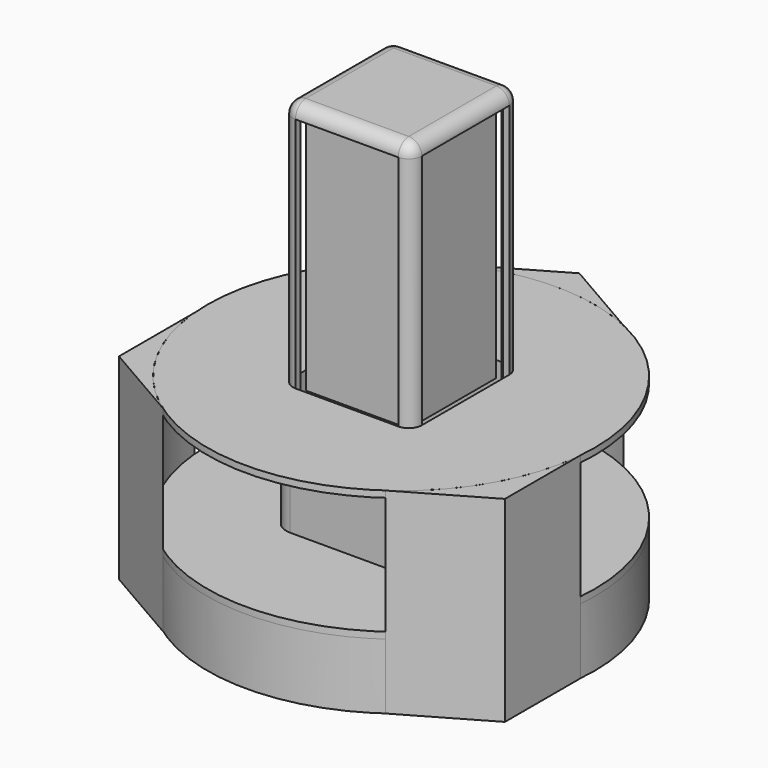
from build123d import *

# Parameters (mm, degrees)
F2_DEPTH     = 76.2
F0_R         = 75.1900139913
F3_DEPTH     = 25.4
F4_W         = 50.0582046807
F4_H         = 52.6002421975
F5_DEPTH     = 147.828
F6_R         = 5.08
F7_DEPTH     = 50.8
F8_T         = -2.54
F9_T         = 2.54
F9_T4_ANGLE  = 90.000000001
F9_T6_ANGLE  = 90.000000001
F9_T8_ANGLE  = 90.000000001
F9_T10_ANGLE = 90.000000001
F10_DEPTH    = 99.822


# Not quite as in the source:
# - a shell that OpenCascade refuses in one call is made with other operations: the cavity is built on its own and cut out


with BuildPart() as f2:
    # F1 (on face) → F2 (new body)
    with BuildSketch(Plane.XY):
        with BuildLine():
            Line((-74.8964771628, -6.6374628139), (-74.8964771628, -43.2415012513))
            Line((-74.8964771628, -43.2415012513), (-43.1964499949, -61.5435204701))
            ThreePointArc((-43.1964499949, -61.5435204701), (-65.1164622274, -37.5950069956), (-74.8964771628, -6.6374628139))
        make_face()
    extrude(amount=F2_DEPTH)


with BuildPart() as f2b:
    # F1 (on face) → F2, piece 2 (new body)
    with BuildSketch(Plane.XY):
        with BuildLine():
            Line((0, 86.4830025026), (-31.7000271679, 68.1809832839))
            ThreePointArc((-31.7000271679, 68.1809832839), (0, 75.1900139913), (31.7000271679, 68.1809832839))
            Line((31.7000271679, 68.1809832839), (0, 86.4830025026))
        make_face()
    extrude(amount=F2_DEPTH)


with BuildPart() as f2c:
    # F1 (on face) → F2, piece 3 (new body)
    with BuildSketch(Plane.XY):
        with BuildLine():
            ThreePointArc((74.8964771628, -6.6374628139), (65.1164622274, -37.5950069956), (43.1964499949, -61.5435204701))
            Line((43.1964499949, -61.5435204701), (74.8964771628, -43.2415012513))
            Line((74.8964771628, -43.2415012513), (74.8964771628, -6.6374628139))
        make_face()
    extrude(amount=F2_DEPTH)


with BuildPart() as f3:
    # F0 (on Top) → F3 (new body)
    with BuildSketch(Plane.XY):
        Circle(F0_R)
    extrude(amount=F3_DEPTH)

    # F4 (on face) → F5 (join)
    with BuildSketch(Plane.XY.offset(25.4)):
        Rectangle(F4_W, F4_H)
    extrude(amount=F5_DEPTH)

    # F6
    f6_edges = [f3.edges().sort_by_distance(p)[0] for p in [
        (25.029102, -26.300121, 99.314),
        (25.029102, 26.300121, 99.314),
        (-25.029102, 26.300121, 99.314),
        (-25.029102, -26.300121, 99.314),
        (-25.029102, 0, 173.228),
        (0, -26.300121, 173.228),
        (0, 26.300121, 173.228),
        (25.029102, 0, 173.228),
    ]]
    fillet(f6_edges, radius=F6_R)


with BuildPart() as f7:
    # F7 (new): a face of the model
    f7_faces = [f3.part.faces().sort_by_distance(p)[0] for p in [
        (27.1557970912, 0, 25.4),
    ]]
    extrude(f7_faces, amount=F7_DEPTH)

    # F8
    f8_openings = [f7.faces().sort_by_distance(p)[0] for p in [
        (-75.190014, 0, 50.8),
    ]]
    offset(amount=F8_T, openings=f8_openings)


with BuildPart() as f3_1:
    add(f3.part)

    # F9: shell of thickness 2.54, made by hand


with BuildPart() as f9_core1:
    # F9_t2: copy of F3
    add(f3_1.part)

    # the walls: a layer under each face that stays
    f9_faces = [f9_core1.faces().sort_by_distance(p)[0] for p in [
        (-50.1266759942, -50.1266759942, 25.4),
        (23.5412047888, -24.8122235472, 96.774),
        (23.5412047888, 24.8122235472, 96.774),
        (-23.5412047888, -24.8122235472, 96.774),
        (-23.5412047888, 24.8122235472, 96.774),
        (-75.1900139913, 0, 12.7),
        (23.5412047888, 0, 171.7401024484),
        (22.4891023403, -23.7601210988, 171.7401024484),
        (22.4891023403, 23.7601210988, 171.7401024484),
        (0, -24.8122235472, 171.7401024484),
        (0, 24.8122235472, 171.7401024484),
        (-22.4891023403, -23.7601210988, 171.7401024484),
        (-22.4891023403, 23.7601210988, 171.7401024484),
        (-23.5412047888, 0, 171.7401024484),
        (0, 0, 0),
        (0, 0, 173.228),
    ]]
    thicken(f9_faces, amount=-F9_T, mode=Mode.SUBTRACT)

    # F9_s3 → F9_t4 (revolve, cut)
    with BuildSketch(Plane.XZ.offset(21.2201210988)):
        Polygon((25.0545023403, 25.4254), (25.0291023403, 22.86), (22.4891023403, 22.86), (22.4891023403, 25.4), align=None)
    revolve(axis=Axis((19.9491023403, -21.2201210988, 25.4), (0, 0, -1)), revolution_arc=F9_T4_ANGLE, mode=Mode.SUBTRACT)

    # F9_s5 → F9_t6 (revolve, cut)
    with BuildSketch(Plane.XZ.offset(-21.2201210988)):
        Polygon((25.0545023403, 25.4254), (25.0291023403, 22.86), (22.4891023403, 22.86), (22.4891023403, 25.4), align=None)
    revolve(axis=Axis((19.9491023403, 21.2201210988, 25.4), (0, 0, 1)), revolution_arc=F9_T6_ANGLE, mode=Mode.SUBTRACT)

    # F9_s7 → F9_t8 (revolve, cut)
    with BuildSketch(Plane.XZ.offset(21.2201210988)):
        Polygon((-25.0545023403, 25.4254), (-25.0291023403, 22.86), (-22.4891023403, 22.86), (-22.4891023403, 25.4), align=None)
    revolve(axis=Axis((-19.9491023403, -21.2201210988, 25.4), (0, 0, 1)), revolution_arc=F9_T8_ANGLE, mode=Mode.SUBTRACT)

    # F9_s9 → F9_t10 (revolve, cut)
    with BuildSketch(Plane.YZ.offset(-19.9491023403)):
        Polygon((26.3255210988, 25.4254), (26.3001210988, 22.86), (23.7601210988, 22.86), (23.7601210988, 25.4), align=None)
    revolve(axis=Axis((-19.9491023403, 21.2201210988, 25.4), (0, 0, 1)), revolution_arc=F9_T10_ANGLE, mode=Mode.SUBTRACT)


with BuildPart() as f3_2:
    add(f3_1.part)

    # what is left inside the walls is the cavity
    f9_cavity = [f9_core1.part.solids().sort_by_distance(p)[0] for p in [
        (0, -24.216671, 2.5654),
    ]]
    add(f9_cavity, mode=Mode.SUBTRACT)

    # F10 (add): a face of the model
    f10_faces = [f3_2.faces().sort_by_distance(p)[0] for p in [
        (0, 0, 173.228),
    ]]
    extrude(f10_faces, amount=-F10_DEPTH)


solid = Compound([f2.part, f2b.part, f2c.part, f7.part, f3_2.part])
